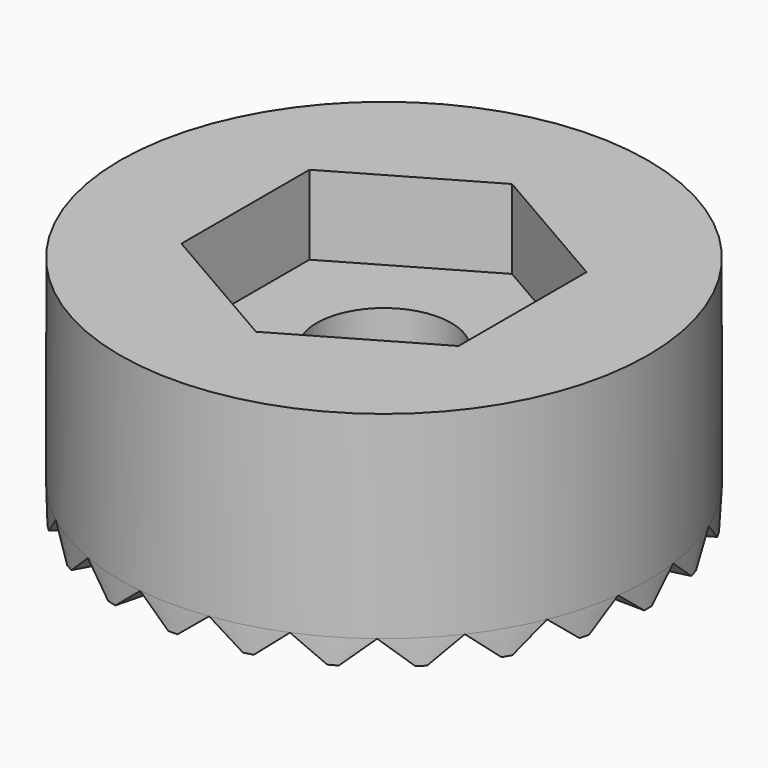
from build123d import *

# Parameters (mm, degrees)
F0_R            = 2.159
F1_DEPTH        = 3.81
F0_R_2          = 8.4666666667
F2_DEPTH        = 6.35
F6_COPIES_COUNT = 24


# Not quite as in the source:
# - a pattern or mirror of a feature is missing from the dataset's text; its kind, count and spacing are read off the source's solid


with BuildPart() as f1:
    # F0 (on Top) → F1 (new body)
    with BuildSketch(Plane.XY):
        Polygon((4.445, -2.5663219465), (4.445, 2.5663219465), (0, 5.1326438931), (-4.445, 2.5663219465), (-4.445, -2.5663219465), (0, -5.1326438931), align=None)
        Circle(F0_R, mode=Mode.SUBTRACT)
    extrude(amount=F1_DEPTH)

    # F0 (on Top) → F2 (join)
    with BuildSketch(Plane.XY):
        Circle(F0_R_2)
        Polygon((0, 5.1326438931), (4.445, 2.5663219465), (4.445, -2.5663219465), (0, -5.1326438931), (-4.445, -2.5663219465), (-4.445, 2.5663219465), align=None, mode=Mode.SUBTRACT)
    extrude(amount=F2_DEPTH)

    # F3 (on face) → F6 section 0
    with BuildSketch(Plane.XY):
        with BuildLine():
            Line((0.7459571885, 5.6661073828), (1.1051217608, 8.3942331596))
            ThreePointArc((1.1051217608, 8.3942331596), (0, 8.4666666667), (-1.1051217608, 8.3942331596))
            Line((-1.1051217608, 8.3942331596), (-0.7459571885, 5.6661073828))
            ThreePointArc((-0.7459571885, 5.6661073828), (0, 5.715), (0.7459571885, 5.6661073828))
        make_face()
    # F5 (on offset) → F6 section 1
    with BuildSketch(Plane.XY.offset(-0.79375)):
        with BuildLine():
            Line((0.0997405028, 5.7141295778), (0.1477637078, 8.4653771523))
            ThreePointArc((0.1477637078, 8.4653771523), (0, 8.4666666667), (-0.1477637078, 8.4653771523))
            Line((-0.1477637078, 8.4653771523), (-0.0997405028, 5.7141295778))
            ThreePointArc((-0.0997405028, 5.7141295778), (0, 5.715), (0.0997405028, 5.7141295778))
        make_face()
    f6 = loft()

    # F6_copies: F6 ×24 about axis
    f6_copies_axis = Axis((0, 0, 0), (0, 0, 1))
    for i in range(1, F6_COPIES_COUNT):
        add(f6.rotate(f6_copies_axis, i * 360 / F6_COPIES_COUNT))


solid = f1.part
